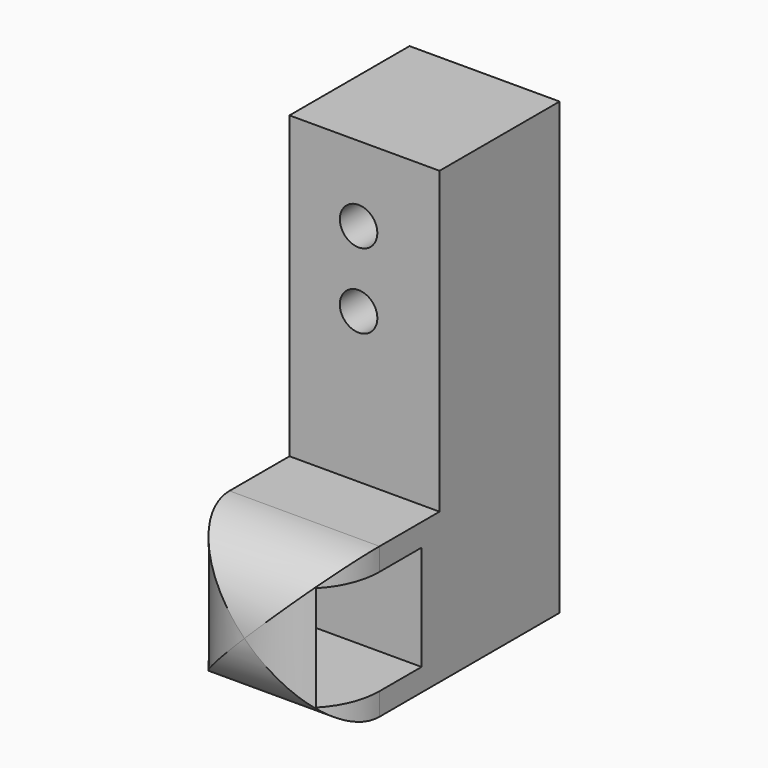
from build123d import *

# Parameters (mm, degrees)
F0_W        = 25.4
F0_H        = 76.2
F0_R        = 3.175
F1_DEPTH    = 25.4
F2_W        = 25.4
F2_H        = 25.4
F3_DEPTH    = 25.4
F4_W        = 17.78
F4_H        = 17.78
F5_DEPTH    = 63.5
F6_T1_DEPTH = 88.9
F6_T3_DEPTH = 88.9


# Not quite as in the source:
# - a fillet or chamfer that OpenCascade refuses, or shapes differently, is made with other operations: its cross-section is extruded or revolved along the edge and cut away or added


with BuildPart() as f1:
    # F0 (on Front) → F1 (new body)
    with BuildSketch(Plane.XZ):
        with Locations((1.0031497249, 16.5614479933)):
            Rectangle(F0_W, F0_H)
        with Locations((0, 29.2614479933)):
            Circle(F0_R, mode=Mode.SUBTRACT)
        with Locations((0, 41.9614479933)):
            Circle(F0_R, mode=Mode.SUBTRACT)
    extrude(amount=F1_DEPTH)

    # F2 (on face) → F3 (join)
    with BuildSketch(Plane.XZ.offset(25.4)):
        with Locations((1.0031497249, -8.8385520067)):
            Rectangle(F2_W, F2_H)
    extrude(amount=F3_DEPTH)

    # F4 (on face) → F5 (cut, symmetric)
    with BuildSketch(Plane(origin=(-11.6968502751, 0, 0), x_dir=(0, -1, 0), z_dir=(-1, 0, 0))):
        with Locations((38.1, -8.8385520067)):
            Rectangle(F4_W, F4_H)
    extrude(amount=F5_DEPTH, both=True, mode=Mode.SUBTRACT)

    # F6: fillet of radius 12.7 on 4 edges, made by hand

    # F6_s2 → F6_t1 (cut)
    with BuildSketch(Plane.YZ.offset(-43.4468502751)):
        with BuildLine():
            ThreePointArc((-50.8, -8.8385520067), (-47.0802561211, 0.1417041144), (-38.1, 3.8614479933))
            Line((-38.1, 3.8614479933), (-50.8, 3.8614479933))
            Line((-50.8, 3.8614479933), (-50.8, -8.8385520067))
        make_face()
        with BuildLine():
            ThreePointArc((-38.1, -21.5385520067), (-47.0802561211, -17.8188081278), (-50.8, -8.8385520067))
            Line((-50.8, -8.8385520067), (-50.8, -21.5385520067))
            Line((-50.8, -21.5385520067), (-38.1, -21.5385520067))
        make_face()
    extrude(amount=F6_T1_DEPTH, mode=Mode.SUBTRACT)

    # F6_s4 → F6_t3 (cut)
    with BuildSketch(Plane.XY.offset(-53.2885520067)):
        with BuildLine():
            ThreePointArc((1.0031497249, -50.8), (-7.9771063962, -47.0802561211), (-11.6968502751, -38.1))
            Line((-11.6968502751, -38.1), (-11.6968502751, -50.8))
            Line((-11.6968502751, -50.8), (1.0031497249, -50.8))
        make_face()
        with BuildLine():
            ThreePointArc((13.7031497249, -38.1), (9.983405846, -47.0802561211), (1.0031497249, -50.8))
            Line((1.0031497249, -50.8), (13.7031497249, -50.8))
            Line((13.7031497249, -50.8), (13.7031497249, -38.1))
        make_face()
    extrude(amount=F6_T3_DEPTH, mode=Mode.SUBTRACT)


solid = f1.part
